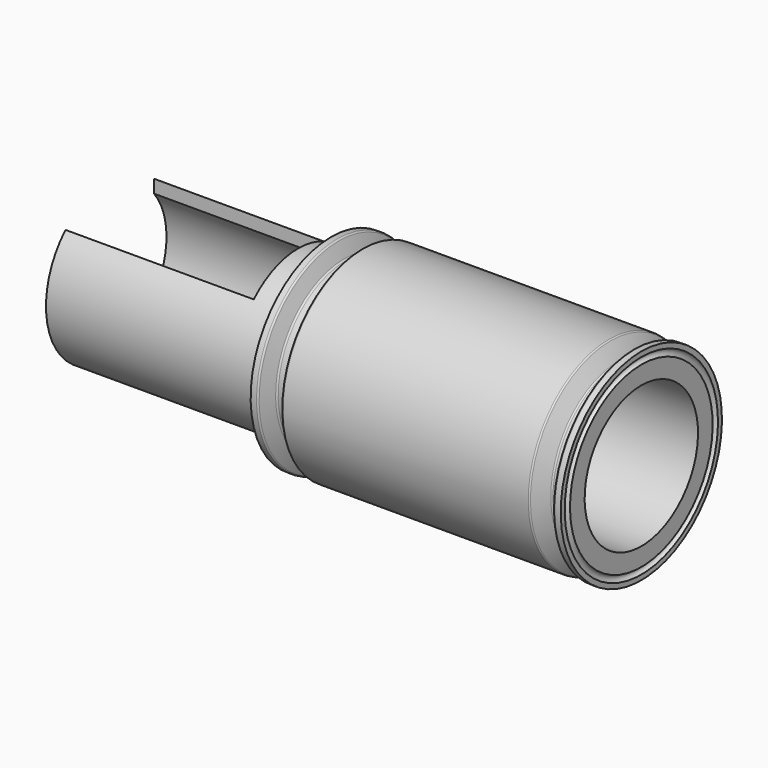
from build123d import *

# Parameters (mm, degrees)
F3_R        = 21.5
F4_DEPTH    = 25
F6_W        = 85
F6_H        = 50
F7_DEPTH    = 30
F8_T4_ANGLE = 73.3070095704
F8_T9_ANGLE = 73.3070095704
F9_R        = 5
F10_DEPTH   = 50


# Not quite as in the source:
# - a fillet or chamfer that OpenCascade refuses, or shapes differently, is made with other operations: its cross-section is extruded or revolved along the edge and cut away or added


with BuildPart() as f1:
    # F0 (on Front) → F1 (revolve)
    with BuildSketch(Plane.XZ):
        with BuildLine():
            Line((-240, 36), (-240, 32))
            Line((-240, 32), (0, 32))
            Line((0, 32), (0, 40.25))
            ThreePointArc((0, 40.25), (-1.5, 41.75), (0, 43.25))
            Line((0, 43.25), (0, 45.5))
            Line((0, 45.5), (-2.6398339694, 45.5))
            ThreePointArc((-2.6398339694, 45.5), (-3.0986951185, 45.3553216354), (-3.3915880661, 44.9736161147))
            Line((-3.3915880661, 44.9736161147), (-5.7199901792, 38.5763838853))
            ThreePointArc((-5.7199901792, 38.5763838853), (-6.0128831268, 38.1946783646), (-6.4717442759, 38.05))
            Line((-6.4717442759, 38.05), (-9.4496980299, 38.05))
            ThreePointArc((-9.4496980299, 38.05), (-9.8496980299, 38.157179677), (-10.142518353, 38.45))
            Line((-10.142518353, 38.45), (-13.9818976431, 45.1))
            ThreePointArc((-13.9818976431, 45.1), (-14.2747179661, 45.392820323), (-14.6747179661, 45.5))
            Line((-14.6747179661, 45.5), (-125.3252820339, 45.5))
            ThreePointArc((-125.3252820339, 45.5), (-125.7252820339, 45.392820323), (-126.0181023569, 45.1))
            Line((-126.0181023569, 45.1), (-129.857481647, 38.45))
            ThreePointArc((-129.857481647, 38.45), (-130.1503019701, 38.157179677), (-130.5503019701, 38.05))
            Line((-130.5503019701, 38.05), (-133.5282557241, 38.05))
            ThreePointArc((-133.5282557241, 38.05), (-133.9871168732, 38.1946783646), (-134.2800098208, 38.5763838853))
            Line((-134.2800098208, 38.5763838853), (-136.6084119339, 44.9736161147))
            ThreePointArc((-136.6084119339, 44.9736161147), (-136.9013048815, 45.3553216354), (-137.3601660306, 45.5))
            Line((-137.3601660306, 45.5), (-140, 45.5))
            Line((-140, 45.5), (-140, 43.25))
            ThreePointArc((-140, 43.25), (-138.5, 41.75), (-140, 40.25))
            Line((-140, 40.25), (-140, 36))
            Line((-140, 36), (-240, 36))
        make_face()
    revolve(axis=Axis((-38.3716828611, 0, 0), (-1, 0, 0)))

    # F3 (on offset) → F4 (cut)
    with BuildSketch(Plane.XY.offset(-45.5)):
        with Locations((-88.5, 0)):
            Circle(F3_R)
    extrude(amount=F4_DEPTH, mode=Mode.SUBTRACT)

    # F6 (on offset) → F7 (cut)
    with BuildSketch(Plane.XY.offset(45.5)):
        with Locations((-197.5, 0)):
            Rectangle(F6_W, F6_H)
    extrude(amount=-F7_DEPTH, mode=Mode.SUBTRACT)

    # F8: fillet of radius 5 on 2 edges, made by hand


with BuildPart() as f8_tool2:
    # F8_s3 → F8_t4 (revolve)
    with BuildSketch(Plane.XZ):
        with BuildLine():
            ThreePointArc((-155, 36), (-153.2632981746, 33.1270166538), (-150.1010205144, 32))
            Line((-150.1010205144, 32), (-155, 32))
            Line((-155, 32), (-155, 36))
        make_face()
    revolve(axis=Axis((-155, 0, 0), (1, 0, 0)), revolution_arc=F8_T4_ANGLE)

    split(bisect_by=Plane.XZ.offset(25), keep=Keep.BOTTOM)


with BuildPart() as f1_1:
    add(f1.part)

    # F8_t1: cut F8_tool2
    add(f8_tool2.part, mode=Mode.SUBTRACT)


with BuildPart() as f8_tool7:
    # F8_s8 → F8_t9 (revolve)
    with BuildSketch(Plane(origin=(0, 0, 0), x_dir=(1, 0, 0), z_dir=(0, 0.2872433376, -0.9578576434))):
        with BuildLine():
            ThreePointArc((-155, -36), (-153.2632981746, -33.1270166538), (-150.1010205144, -32))
            Line((-150.1010205144, -32), (-155, -32))
            Line((-155, -32), (-155, -36))
        make_face()
    revolve(axis=Axis((-155, 0, 0), (1, 0, 0)), revolution_arc=F8_T9_ANGLE)

    split(bisect_by=Plane.XZ.offset(-25), keep=Keep.TOP)


with BuildPart() as f1_2:
    add(f1_1.part)

    # F8_t6: cut F8_tool7
    add(f8_tool7.part, mode=Mode.SUBTRACT)

    # F9 (on offset) → F10 (cut)
    with BuildSketch(Plane.XY.offset(-45.5)):
        with Locations((-40, 0)):
            Circle(F9_R)
    extrude(amount=F10_DEPTH, mode=Mode.SUBTRACT)


solid = f1_2.part
